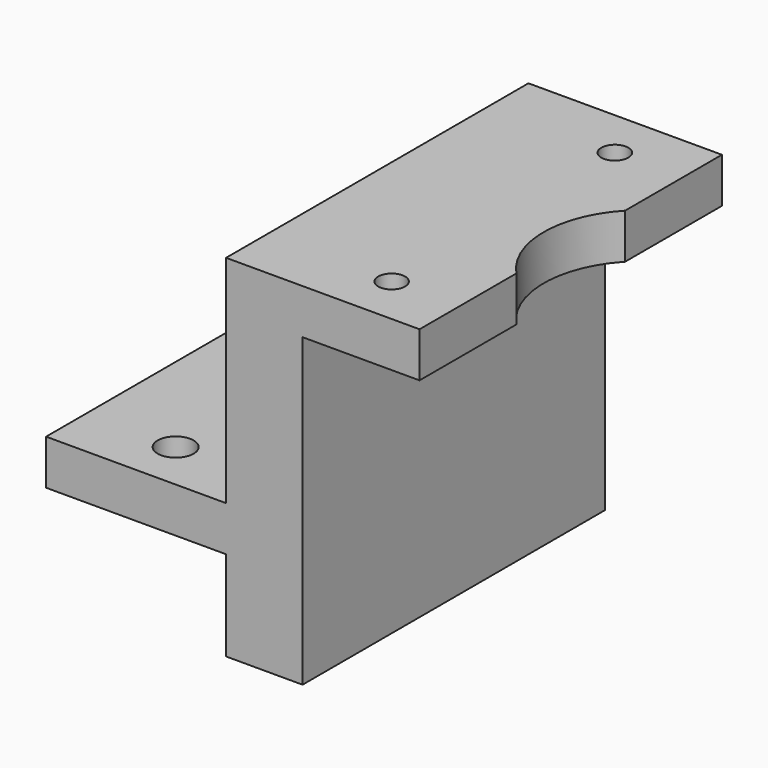
from build123d import *

# Parameters (mm, degrees)
F0_W          = 20
F0_H          = 42
F0_R          = 2
F1_DEPTH      = 5
F0_W_2        = 8.5
F2_DEPTH      = 29
F2_DEPTH_BACK = 10
F0_R_2        = 1.5
F3_DEPTH      = 29
F4_DEPTH      = 24


# Not quite as in the source:
# - a feature names something its author has since deleted; it is built from what else it names


with BuildPart() as f1:
    # F0 (on Top) → F1 (new body)
    with BuildSketch(Plane.XY):
        with Locations((-2.5607131049, 21)):
            Rectangle(F0_W, F0_H)
        with Locations((-2.5607131049, 5.5)):
            Circle(F0_R, mode=Mode.SUBTRACT)
        with Locations((-2.5607131049, 36.5)):
            Circle(F0_R, mode=Mode.SUBTRACT)
    extrude(amount=F1_DEPTH)

    # F0 (on Top) → F2 (join, two sides)
    with BuildSketch(Plane.XY) as f2_sk:
        with Locations((11.6892868951, 21)):
            Rectangle(F0_W_2, F0_H)
    extrude(amount=F2_DEPTH)
    extrude(f2_sk.sketch, amount=-F2_DEPTH_BACK)

    # F0 (on Top) → F3 (join)
    with BuildSketch(Plane.XY):
        with BuildLine():
            ThreePointArc((28.9392868951, 13.4501655647), (25.9392868951, 21), (28.9392868951, 28.5498344353))
            Line((28.9392868951, 28.5498344353), (28.9392868951, 42))
            Line((28.9392868951, 42), (15.9392868951, 42))
            Line((15.9392868951, 42), (15.9392868951, 0))
            Line((15.9392868951, 0), (28.9392868951, 0))
            Line((28.9392868951, 0), (28.9392868951, 13.4501655647))
        make_face()
        with Locations((21.4392868951, 5.5)):
            Circle(F0_R_2, mode=Mode.SUBTRACT)
        with Locations((21.4392868951, 36.5)):
            Circle(F0_R_2, mode=Mode.SUBTRACT)
    extrude(amount=F3_DEPTH)

    # F0 (on Top) → F4 (cut)
    with BuildSketch(Plane.XY):
        with BuildLine():
            ThreePointArc((28.9392868951, 13.4501655647), (25.9392868951, 21), (28.9392868951, 28.5498344353))
            Line((28.9392868951, 28.5498344353), (28.9392868951, 42))
            Line((28.9392868951, 42), (15.9392868951, 42))
            Line((15.9392868951, 42), (15.9392868951, 0))
            Line((15.9392868951, 0), (28.9392868951, 0))
            Line((28.9392868951, 0), (28.9392868951, 13.4501655647))
        make_face()
        with Locations((21.4392868951, 5.5)):
            Circle(F0_R_2, mode=Mode.SUBTRACT)
        with Locations((21.4392868951, 36.5)):
            Circle(F0_R_2, mode=Mode.SUBTRACT)
    extrude(amount=F4_DEPTH, mode=Mode.SUBTRACT)


solid = f1.part
